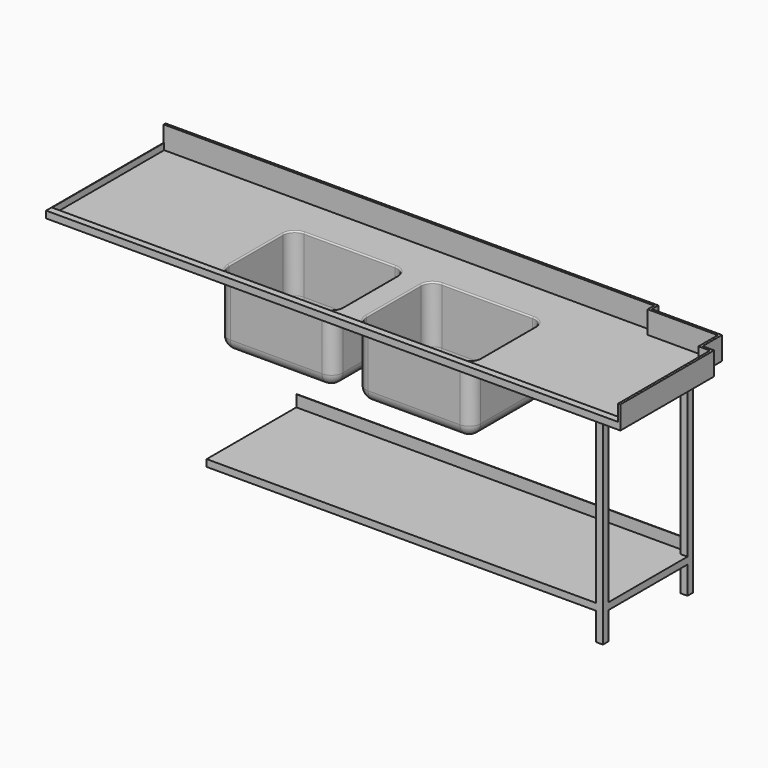
from build123d import *

# Parameters (mm, degrees)
F1_DEPTH     = 100
F3_DEPTH     = 98
F4_W         = 500
F4_H         = 400
F5_DEPTH     = 300
F6_W         = 2490
F6_H         = 30
F7_DEPTH     = 70
F8_T         = 2
F8_T3_DEPTH  = 104
F8_T5_DEPTH  = 34
F8_T7_DEPTH  = 32
F8_T9_DEPTH  = 102
F8_T11_DEPTH = 504
F8_T13_DEPTH = 404
F8_T15_DEPTH = 504
F9_R         = 50
F10_R        = 25
F11_DEPTH    = 2
F12_W        = 30
F12_H        = 30
F13_DEPTH    = 865
F14_R        = 6
F15_W        = 2
F15_H        = 28
F16_DEPTH    = 610
F18_DEPTH    = 1725


# Not quite as in the source:
# - a shell that OpenCascade refuses in one call is made with other operations: the cavity is built on its own and cut out
# - a feature names something its author has since deleted; it is built from what else it names


with BuildPart() as f1:
    # F0 (on Top) → F1 (new body)
    with BuildSketch(Plane.XY):
        Polygon((0, 650), (0, 0), (2500, 0), (2500, 510), (2450, 510), (2450, 615), (2145, 615), (2145, 650), align=None)
    extrude(amount=F1_DEPTH)

    # F2 (on face) → F3 (cut)
    with BuildSketch(Plane.XY.offset(100)):
        Polygon((0, 640), (0, 30), (2490, 30), (2490, 500), (2440, 500), (2440, 605), (2135, 605), (2135, 640), align=None)
    extrude(amount=-F3_DEPTH, mode=Mode.SUBTRACT)

    # F4 (on face) → F5 (join)
    with BuildSketch(Plane.XY.offset(2)):
        with Locations((950, 265)):
            Rectangle(F4_W, F4_H)
        with Locations((1550, 265)):
            Rectangle(F4_W, F4_H)
    extrude(amount=-F5_DEPTH)

    # F6 (on face) → F7 (cut)
    with BuildSketch(Plane.XY.offset(100)):
        with Locations((1245, 15)):
            Rectangle(F6_W, F6_H)
    extrude(amount=-F7_DEPTH, mode=Mode.SUBTRACT)

    # F8: shell of thickness 2, made by hand


with BuildPart() as f8_core1:
    # F8_t2: copy of F1
    add(f1.part)

    # the walls: a layer under each face that stays
    f8_faces = [f8_core1.faces().sort_by_distance(p)[0] for p in [
        (0, 21.6666666667, 23.3333333333),
        (1072.5, 650, 50),
        (2145, 632.5, 50),
        (2297.5, 615, 50),
        (2450, 562.5, 50),
        (2475, 510, 50),
        (2500, 255, 50),
        (97.65625, 641.975308642, 100),
        (2490, 250, 51),
        (2465, 500, 51),
        (2440, 552.5, 51),
        (2287.5, 605, 51),
        (2135, 622.5, 51),
        (1067.5, 640, 51),
        (1245, 30, 16),
        (1245, 15, 30),
        (416.6666666667, 0, 16.6666666667),
        (1250, 325, 0),
        (1800, 265, -149),
        (1550, 265, -298),
        (1550, 65, -149),
        (1300, 265, -149),
        (1550, 465, -149),
        (1200, 265, -149),
        (950, 265, -298),
        (950, 65, -149),
        (700, 265, -149),
        (950, 465, -149),
    ]]
    thicken(f8_faces, amount=-F8_T, mode=Mode.SUBTRACT)

    # F8_s4 → F8_t3 (cut)
    with BuildSketch(Plane.XY.offset(-2)):
        Polygon((2145.02, 615.02), (2143, 615), (2143, 613), (2145, 613), align=None)
        Polygon((2450.02, 510.02), (2448, 510), (2448, 508), (2450, 508), align=None)
    extrude(amount=F8_T3_DEPTH, mode=Mode.SUBTRACT)

    # F8_s6 → F8_t5 (cut)
    with BuildSketch(Plane.XZ.offset(-32)):
        Polygon((2489.98, 30.02), (2492, 30), (2492, 28), (2490, 28), align=None)
    extrude(amount=F8_T5_DEPTH, mode=Mode.SUBTRACT)

    # F8_s8 → F8_t7 (cut)
    with BuildSketch(Plane.XY):
        Polygon((2489.98, 30.02), (2492, 30), (2492, 28), (2490, 28), align=None)
    extrude(amount=F8_T7_DEPTH, mode=Mode.SUBTRACT)

    # F8_s10 → F8_t9 (cut)
    with BuildSketch(Plane.XY):
        Polygon((2489.98, 499.98), (2492, 500), (2492, 502), (2490, 502), align=None)
        Polygon((2439.98, 604.98), (2442, 605), (2442, 607), (2440, 607), align=None)
        Polygon((2134.98, 639.98), (2137, 640), (2137, 642), (2135, 642), align=None)
    extrude(amount=F8_T9_DEPTH, mode=Mode.SUBTRACT)

    # F8_s12 → F8_t11 (cut)
    with BuildSketch(Plane.YZ.offset(698)):
        Polygon((465.02, -0.02), (465, 2), (463, 2), (463, 0), align=None)
        Polygon((64.98, -0.02), (65, 2), (67, 2), (67, 0), align=None)
    extrude(amount=F8_T11_DEPTH, mode=Mode.SUBTRACT)

    # F8_s14 → F8_t13 (cut)
    with BuildSketch(Plane.XZ.offset(-467)):
        Polygon((699.98, -0.02), (700, 2), (702, 2), (702, 0), align=None)
        Polygon((1200.02, -0.02), (1200, 2), (1198, 2), (1198, 0), align=None)
        Polygon((1299.98, -0.02), (1300, 2), (1302, 2), (1302, 0), align=None)
        Polygon((1800.02, -0.02), (1800, 2), (1798, 2), (1798, 0), align=None)
    extrude(amount=F8_T13_DEPTH, mode=Mode.SUBTRACT)

    # F8_s16 → F8_t15 (cut)
    with BuildSketch(Plane.YZ.offset(1298)):
        Polygon((465.02, -0.02), (465, 2), (463, 2), (463, 0), align=None)
        Polygon((64.98, -0.02), (65, 2), (67, 2), (67, 0), align=None)
    extrude(amount=F8_T15_DEPTH, mode=Mode.SUBTRACT)


with BuildPart() as f1_1:
    add(f1.part)

    # what is left inside the walls is the cavity
    f8_cavity = [f8_core1.part.solids().sort_by_distance(p)[0] for p in [
        (1072.5, 647.98, 66),
        (950, 199, -295.98),
        (1550, 199, -295.98),
    ]]
    add(f8_cavity, mode=Mode.SUBTRACT)

    # F9
    f9_edges = [f1_1.edges().sort_by_distance(p)[0] for p in [
        (702, 463, -147),
        (1198, 463, -147),
        (950, 463, -296),
        (702, 67, -147),
        (1198, 67, -147),
        (1198, 265, -296),
        (950, 67, -296),
        (702, 265, -296),
        (1302, 265, -296),
        (1302, 463, -147),
        (1550, 463, -296),
        (1798, 463, -147),
        (1798, 265, -296),
        (1798, 67, -147),
        (1550, 67, -296),
        (1302, 67, -147),
        (700, 65, -149),
        (700, 265, -298),
        (950, 65, -298),
        (1300, 65, -149),
        (1300, 265, -298),
        (1550, 65, -298),
        (1200, 65, -149),
        (1200, 265, -298),
        (1800, 65, -149),
        (1800, 265, -298),
        (1800, 465, -149),
        (1550, 465, -298),
        (1300, 465, -149),
        (1200, 465, -149),
        (950, 465, -298),
        (700, 465, -149),
    ]]
    fillet(f9_edges, radius=F9_R)

    # F10 (on face) → F11 (cut, through all)
    with BuildSketch(Plane.XY.offset(-296)):
        with Locations((1048, 313)):
            Circle(F10_R)
        with Locations((1648, 313)):
            Circle(F10_R)
    extrude(amount=-F11_DEPTH, mode=Mode.SUBTRACT)

    # F12 (on face) → F13 (join)
    with BuildSketch(Plane(origin=(0, 0, 0), x_dir=(1, 0, 0), z_dir=(0, 0, -1))):
        with Locations((2385, -505)):
            Rectangle(F12_W, F12_H)
        with Locations((2385, -45)):
            Rectangle(F12_W, F12_H)
    extrude(amount=F13_DEPTH)

    # F14
    f14_edges = [f1_1.edges().sort_by_distance(p)[0] for p in [
        (950, 463, 2),
        (716.644661, 448.355339, 2),
        (1183.355339, 448.355339, 2),
        (702, 265, 2),
        (1198, 265, 2),
        (716.644661, 81.644661, 2),
        (1183.355339, 81.644661, 2),
        (950, 67, 2),
        (1550, 463, 2),
        (1316.644661, 448.355339, 2),
        (1783.355339, 448.355339, 2),
        (1302, 265, 2),
        (1798, 265, 2),
        (1316.644661, 81.644661, 2),
        (1783.355339, 81.644661, 2),
        (1550, 67, 2),
    ]]
    fillet(f14_edges, radius=F14_R)

    # F15 (on face) → F16 (join, through all)
    with BuildSketch(Plane(origin=(0, 30, 0), x_dir=(-1, 0, 0), z_dir=(0, 1, 0))):
        with Locations((-1, 16)):
            Rectangle(F15_W, F15_H)
    extrude(amount=F16_DEPTH)

    # F17 (on face) → F18 (join)
    with BuildSketch(Plane.YZ.offset(2400)):
        Polygon((30, -745), (520, -745), (520, -665), (518, -665), (518, -715), (30, -715), align=None)
    extrude(amount=-F18_DEPTH)


solid = f1_1.part
